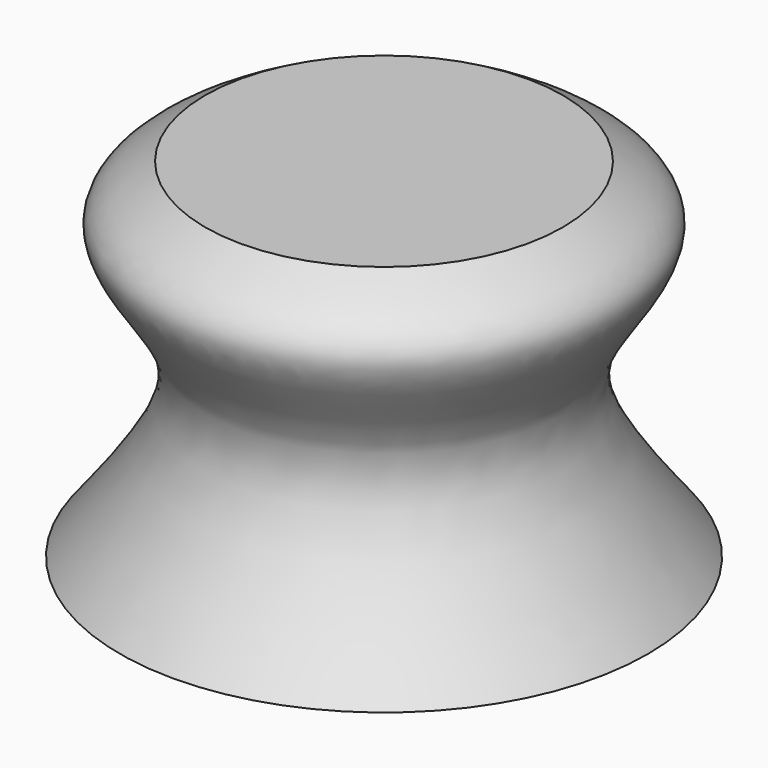
from build123d import *

# Parameters (mm, degrees)
F2_R     = 29.1443160408
F3_DEPTH = 14.732


# Not quite as in the source:
# - a feature names something its author has since deleted; it is built from what else it names


with BuildPart() as f1:
    # F0 (on Front) → F1 (revolve)
    with BuildSketch(Plane.XZ):
        with BuildLine():
            Line((0, 44.0483130515), (-27.9702022672, 44.0483130515))
            add(Edge.make_bspline(
                [(-27.9702022672, 44.0483130515), (-32.3384774692, 41.5807684215), (-42.0960680493, 36.0689155451), (-24.18998033, 19.151376482), (-30.4885813686, 3.3992167823), (-37.5942722132, -5.6593207799), (-41.28934443, -10.3699043393)],
                knots=[0, 0, 0, 0, 0.2198576006, 0.4911046932, 0.7353663492, 1, 1, 1, 1], degree=3))
            Line((-41.28934443, -10.3699043393), (0, -10.3699043393))
            Line((0, -10.3699043393), (0, 44.0483130515))
        make_face()
    revolve(axis=Axis((0, 0, 16.8392043561), (0, 0, -1)))

    # F2 (on face) → F3 (join)
    with BuildSketch(Plane(origin=(0, 0, -10.3699043393), x_dir=(1, 0, 0), z_dir=(0, 0, -1))):
        with Locations((1.5221881913, 0)):
            Circle(F2_R)
    extrude(amount=-F3_DEPTH)


solid = f1.part
